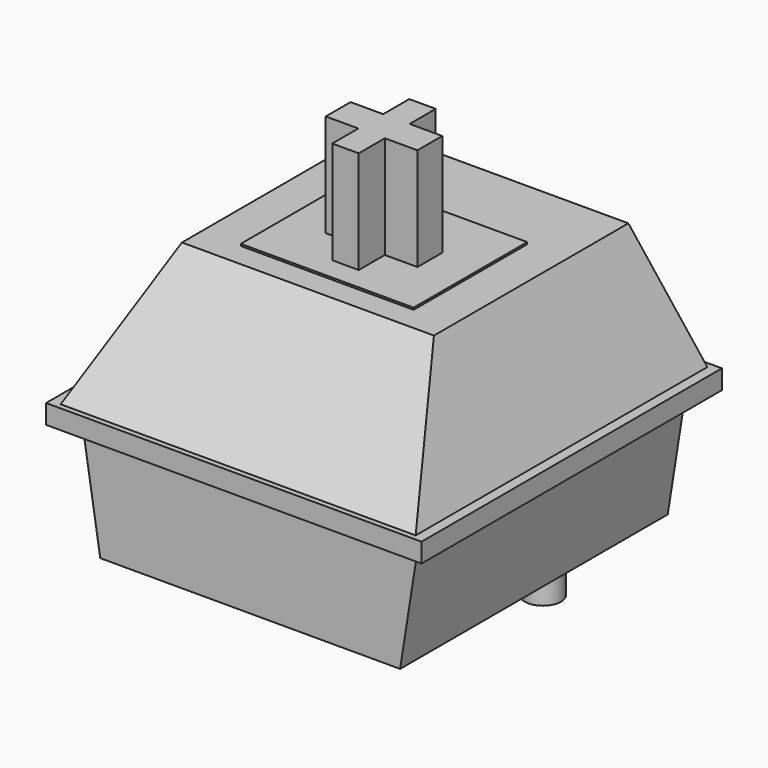
from build123d import *

# Parameters (mm, degrees)
F4_DEPTH       = 10.29
F1_W           = 7.18
F1_H           = 5.9
F5_DEPTH       = 6.02
F1_W_2         = 14.75
F1_H_2         = 15.15
F1_W_3         = 10.47
F1_H_3         = 10.1
F6_DEPTH       = 5.94
F1_W_4         = 15.6
F1_H_4         = 15.6
F7_DEPTH       = 0.8
F8_DEPTH       = 7.801
F8_DEPTH_BACK  = 7.801
F9_DEPTH       = 7.801
F9_DEPTH_BACK  = 7.801
F0_W           = 13.95
F0_H           = 13.9
F0_R           = 0.4953
F0_R_2         = 0.7493
F0_R_3         = 1.9939
F10_DEPTH      = 4.71
F11_DEPTH      = 7.54
F12_DEPTH      = 8.1
F13_DEPTH      = 5.23
F14_DEPTH      = 7.801
F14_DEPTH_BACK = 7.801


with BuildPart() as f4:
    # F1 (on Top) → F4 (new body, through all)
    with BuildSketch(Plane.XY):
        Polygon((0.55, 2), (-0.55, 2), (-0.55, 0.645), (-1.905, 0.645), (-1.905, -0.645), (-0.55, -0.645), (-0.55, -2), (0.55, -2), (0.55, -0.645), (1.905, -0.645), (1.905, 0.645), (0.55, 0.645), align=None)
    extrude(amount=F4_DEPTH)

    # F1 (on Top) → F5 (join, through all)
    with BuildSketch(Plane.XY):
        Rectangle(F1_W, F1_H)
        Polygon((-0.55, 0.645), (-0.55, 2), (0.55, 2), (0.55, 0.645), (1.905, 0.645), (1.905, -0.645), (0.55, -0.645), (0.55, -2), (-0.55, -2), (-0.55, -0.645), (-1.905, -0.645), (-1.905, 0.645), align=None, mode=Mode.SUBTRACT)
    extrude(amount=F5_DEPTH)

    # F1 (on Top) → F6 (join, through all)
    with BuildSketch(Plane.XY):
        Rectangle(F1_W_2, F1_H_2)
        with Locations((0, 1.1)):
            Rectangle(F1_W_3, F1_H_3, mode=Mode.SUBTRACT)
        with Locations((0, 1.1)):
            Rectangle(F1_W_3, F1_H_3)
        Rectangle(F1_W, F1_H, mode=Mode.SUBTRACT)
    extrude(amount=F6_DEPTH)

    # F1 (on Top) → F7 (join, through all)
    with BuildSketch(Plane.XY):
        Rectangle(F1_W_4, F1_H_4)
        Rectangle(F1_W_2, F1_H_2, mode=Mode.SUBTRACT)
    extrude(amount=F7_DEPTH)

    # F2 (on Right) → F8 (cut, two sides)
    with BuildSketch(Plane.YZ) as f8_sk:
        Polygon((-7.8, 5.94), (-7.8, 0.8), (-7.575, 0.8), (-3.95, 5.94), align=None)
        Polygon((6.15, 5.94), (7.575, 0.8), (7.8, 0.8), (7.8, 5.94), align=None)
    extrude(amount=-F8_DEPTH, mode=Mode.SUBTRACT)
    extrude(f8_sk.sketch, amount=F8_DEPTH_BACK, mode=Mode.SUBTRACT)

    # F3 (on Front) → F9 (cut, two sides)
    with BuildSketch(Plane.XZ) as f9_sk:
        Polygon((-7.8, 5.94), (-7.8, 0.8), (-7.375, 0.8), (-5.235, 5.94), align=None)
        Polygon((5.235, 5.94), (7.375, 0.8), (7.8, 0.8), (7.8, 5.94), align=None)
    extrude(amount=-F9_DEPTH, mode=Mode.SUBTRACT)
    extrude(f9_sk.sketch, amount=F9_DEPTH_BACK, mode=Mode.SUBTRACT)

    # F0 (on Top) → F10 (join, through all)
    with BuildSketch(Plane.XY):
        Rectangle(F0_W, F0_H)
        with Locations((-3.81, -5.08)):
            Circle(F0_R, mode=Mode.SUBTRACT)
        with Locations((3.81, -5.08)):
            Circle(F0_R, mode=Mode.SUBTRACT)
        with Locations((-3.81, 2.54)):
            Circle(F0_R_2, mode=Mode.SUBTRACT)
        Circle(F0_R_3, mode=Mode.SUBTRACT)
        with Locations((2.54, 5.08)):
            Circle(F0_R_2, mode=Mode.SUBTRACT)
    extrude(amount=-F10_DEPTH)

    # F0 (on Top) → F11 (join, through all)
    with BuildSketch(Plane.XY):
        Circle(F0_R_3)
    extrude(amount=-F11_DEPTH)

    # F0 (on Top) → F12 (join, through all)
    with BuildSketch(Plane.XY):
        with Locations((-3.81, 2.54)):
            Circle(F0_R_2)
        with Locations((2.54, 5.08)):
            Circle(F0_R_2)
    extrude(amount=-F12_DEPTH)

    # F0 (on Top) → F13 (join, through all)
    with BuildSketch(Plane.XY):
        with Locations((3.81, -5.08)):
            Circle(F0_R)
        with Locations((-3.81, -5.08)):
            Circle(F0_R)
    extrude(amount=-F13_DEPTH)

    # F3 (on Front) → F14 (cut, two sides)
    with BuildSketch(Plane.XZ) as f14_sk:
        Polygon((-6.975, 0), (-7.8, 0), (-7.8, -4.71), (-6.23, -4.71), align=None)
        Polygon((7.8, 0), (6.975, 0), (6.23, -4.71), (7.8, -4.71), align=None)
    extrude(amount=-F14_DEPTH, mode=Mode.SUBTRACT)
    extrude(f14_sk.sketch, amount=F14_DEPTH_BACK, mode=Mode.SUBTRACT)


solid = f4.part
